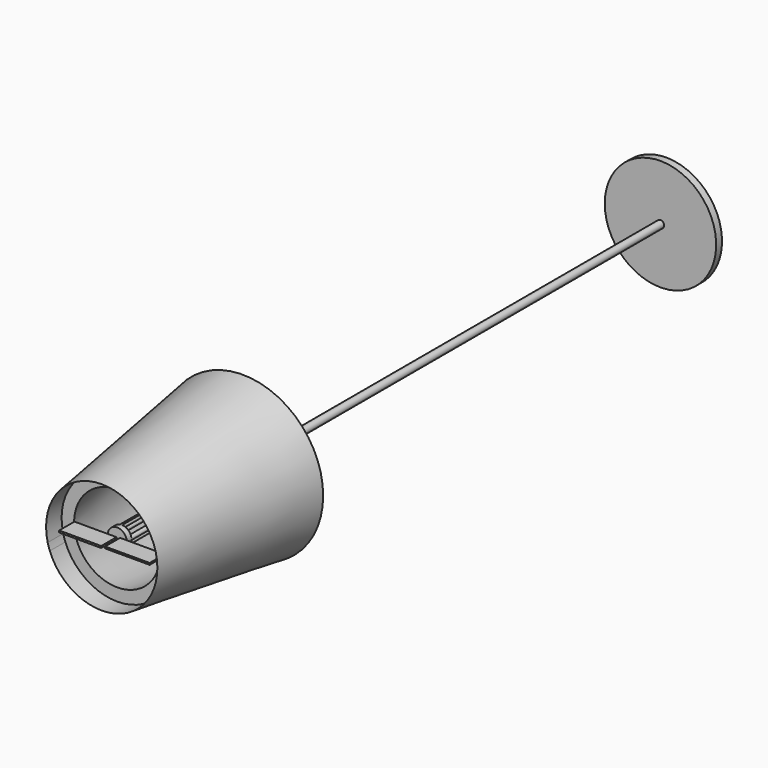
from build123d import *

# Parameters (mm, degrees)
F0_R      = 13.5592595767
F1_DEPTH  = 29.718
F1_TAPER  = 8
F2_T      = -2.54
F3_R      = 1.6206128815
F4_DEPTH  = 1.69587
F5_R      = 0.3642033025
F6_DEPTH  = 25.68642
F7_R      = 0.3599346609
F8_DEPTH  = 25.4
F10_DEPTH = 25.4
F12_DEPTH = 25.4
F14_R     = 1.5374110376
F15_DEPTH = 0.50224
F16_R     = 0.6190660423
F17_DEPTH = 87.54798
F18_R     = 9.3919876404
F18_R_2   = 0.6190660423
F19_DEPTH = 1.23503
F23_DEPTH = 3.27217
F24_W     = 7.0823915303
F24_H     = 0.3065504134
F25_DEPTH = 3.22685
F26_W     = 7.5060166419
F26_H     = 0.2925693989
F27_DEPTH = 3.15669


with BuildPart() as f1:
    # F0 (on Front) → F1 (new body)
    with BuildSketch(Plane.XZ):
        with Locations((-47.4954396486, -26.0666497052)):
            Circle(F0_R)
    extrude(amount=F1_DEPTH, taper=F1_TAPER)

    # F2
    f2_openings = [f1.faces().sort_by_distance(p)[0] for p in [
        (-47.49544, 0, -26.06665),
    ]]
    offset(amount=F2_T, openings=f2_openings, kind=Kind.INTERSECTION)


with BuildPart() as f4:
    # F3 (on face) → F4 (new body)
    with BuildSketch(Plane(origin=(0, -27.178, 0), x_dir=(-1, 0, 0), z_dir=(0, 1, 0))):
        with Locations((47.4954396486, -26.0666497052)):
            Circle(F3_R)
    extrude(amount=F4_DEPTH)

    # F5 (on face) → F6 (join)
    with BuildSketch(Plane(origin=(0, -25.48213, 0), x_dir=(-1, 0, 0), z_dir=(0, 1, 0))):
        with Locations((46.3356487453, -26.1080786586)):
            Circle(F5_R)
    extrude(amount=F6_DEPTH)

    # F7 (on face) → F8 (join)
    with BuildSketch(Plane(origin=(0, -25.48213, 0), x_dir=(-1, 0, 0), z_dir=(0, 1, 0))):
        with Locations((48.4664849937, -26.1451341212)):
            Circle(F7_R)
    extrude(amount=F8_DEPTH)

    # F9 (on face) → F10 (join)
    with BuildSketch(Plane(origin=(0, -25.48213, 0), x_dir=(-1, 0, 0), z_dir=(0, 1, 0))):
        with BuildLine():
            ThreePointArc((47.41794258, -24.4478908238), (47.4240384196, -25.011293234), (47.9109686139, -24.7278176248))
            ThreePointArc((47.9109686139, -24.7278176248), (47.8785730308, -24.5861448369), (47.7878251577, -24.4726306257))
            ThreePointArc((47.7878251577, -24.4726306257), (47.6035935894, -24.4496497557), (47.41794258, -24.4478908238))
        make_face()
    extrude(amount=F10_DEPTH)

    # F11 (on face) → F12 (join)
    with BuildSketch(Plane(origin=(0, -25.48213, 0), x_dir=(-1, 0, 0), z_dir=(0, 1, 0))):
        with BuildLine():
            ThreePointArc((47.1510242573, -27.6502418717), (47.3525978951, -27.5545998612), (47.434509989, -27.347067371))
            ThreePointArc((47.434509989, -27.347067371), (46.9918734087, -27.0767520331), (46.9535594811, -27.5939846375))
            ThreePointArc((46.9535594811, -27.5939846375), (47.0514000406, -27.6252436029), (47.1510242573, -27.6502418717))
        make_face()
    extrude(amount=F12_DEPTH)


with BuildPart() as f15:
    # F14 (on face) → F15 (new body)
    with BuildSketch(Plane(origin=(0, -0.08213, 0), x_dir=(-1, 0, 0), z_dir=(0, 1, 0))):
        with Locations((47.4374033511, -25.9135309607)):
            Circle(F14_R)
    extrude(amount=F15_DEPTH)

    # F16 (on face) → F17 (join)
    with BuildSketch(Plane(origin=(0, 0.42011, 0), x_dir=(-1, 0, 0), z_dir=(0, 1, 0))):
        with Locations((47.4374033511, -25.9135309607)):
            Circle(F16_R)
    extrude(amount=F17_DEPTH)


with BuildPart() as f19:
    # F18 (on face) → F19 (new body)
    with BuildSketch(Plane(origin=(0, 87.96809, 0), x_dir=(-1, 0, 0), z_dir=(0, 1, 0))):
        with Locations((47.4374033511, -25.9135309607)):
            Circle(F18_R)
        with Locations((47.4374033511, -25.9135309607)):
            Circle(F18_R_2, mode=Mode.SUBTRACT)
    extrude(amount=F19_DEPTH)


with BuildPart() as f23_tool:
    # F22 (on face) → F23 (new body)
    with BuildSketch(Plane.XZ.offset(29.718)):
        with BuildLine():
            ThreePointArc((-38.1127725976, -26.0666497052), (-48.6277968924, -16.7525631658), (-56.6047872009, -28.3148107674))
            ThreePointArc((-56.6047872009, -28.3148107674), (-56.4445452516, -28.885388606), (-56.2488679145, -29.4448052056))
            ThreePointArc((-56.2488679145, -29.4448052056), (-45.77731014, -35.2906657493), (-38.1127725976, -26.0666497052))
        make_face()
    extrude(amount=-F23_DEPTH)


with BuildPart() as f1_1:
    add(f1.part)

    # F23: cut by f23_tool
    add(f23_tool.part, mode=Mode.SUBTRACT)


with BuildPart() as f4_1:
    add(f4.part)

    # F23: cut by f23_tool
    add(f23_tool.part, mode=Mode.SUBTRACT)


with BuildPart() as f25:
    # F24 (on face) → F25 (new body)
    with BuildSketch(Plane.XZ.offset(29.718)):
        with Locations((-51.1282850057, -26.0433480144)):
            Rectangle(F24_W, F24_H)
    extrude(amount=-F25_DEPTH)


with BuildPart() as f27:
    # F26 (on face) → F27 (new body)
    with BuildSketch(Plane.XZ.offset(29.718)):
        with Locations((-43.1701745838, -25.8973315358)):
            Rectangle(F26_W, F26_H)
    extrude(amount=-F27_DEPTH)


solid = Compound([f15.part, f19.part, f1_1.part, f4_1.part, f25.part, f27.part])
